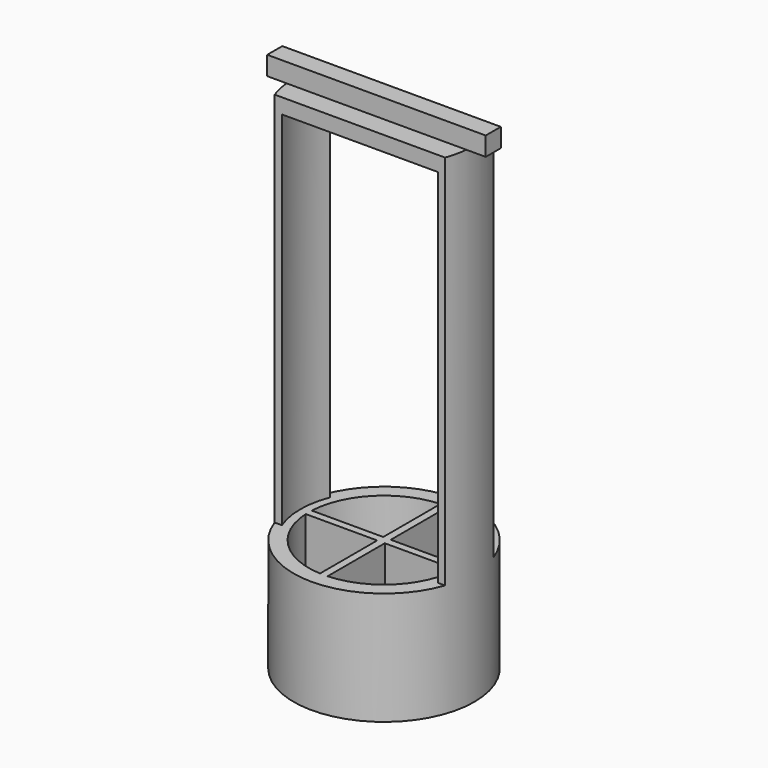
from build123d import *

# Parameters (mm, degrees)
F0_R      = 12
F1_DEPTH  = 15
F3_DEPTH  = 13
F4_R      = 12
F4_R_2    = 11.1
F5_DEPTH  = 50
F7_DEPTH  = 50
F8_W      = 22.627416998
F8_H      = 8
F9_DEPTH  = 2
F10_W     = 29
F10_H     = 2.5
F11_DEPTH = 2.5


with BuildPart() as f1:
    # F0 (on Top) → F1 (new body)
    with BuildSketch(Plane.XY):
        Circle(F0_R)
    extrude(amount=F1_DEPTH)

    # F2 (on face) → F3 (cut)
    with BuildSketch(Plane.XY.offset(15)):
        with BuildLine():
            Line((-0.5, 0.5), (-0.5, 9.9874921777))
            ThreePointArc((-0.5, 9.9874921777), (-7.0710678119, 7.0710678119), (-9.9874921777, 0.5))
            Line((-9.9874921777, 0.5), (-0.5, 0.5))
        make_face()
        with BuildLine():
            Line((0.5, 0.5), (9.9874921777, 0.5))
            ThreePointArc((9.9874921777, 0.5), (7.0710678119, 7.0710678119), (0.5, 9.9874921777))
            Line((0.5, 9.9874921777), (0.5, 0.5))
        make_face()
        with BuildLine():
            ThreePointArc((0.5, -9.9874921777), (7.0710678119, -7.0710678119), (9.9874921777, -0.5))
            Line((9.9874921777, -0.5), (0.5, -0.5))
            Line((0.5, -0.5), (0.5, -9.9874921777))
        make_face()
        with BuildLine():
            ThreePointArc((-9.9874921777, -0.5), (-7.0710678119, -7.0710678119), (-0.5, -9.9874921777))
            Line((-0.5, -9.9874921777), (-0.5, -0.5))
            Line((-0.5, -0.5), (-9.9874921777, -0.5))
        make_face()
    extrude(amount=-F3_DEPTH, mode=Mode.SUBTRACT)

    # F4 (on face) → F5 (join)
    with BuildSketch(Plane.XY.offset(15)):
        Circle(F4_R)
        Circle(F4_R_2, mode=Mode.SUBTRACT)
    extrude(amount=F5_DEPTH)

    # F6 (on face) → F7 (cut)
    with BuildSketch(Plane.XY.offset(65)):
        with BuildLine():
            Line((14.9746745975, -4), (14.8116537966, -4))
            Line((14.8116537966, -4), (11.313708499, -4))
            ThreePointArc((11.313708499, -4), (0, -12), (-11.313708499, -4))
            Line((-11.313708499, -4), (-14.8116537966, -4))
            Line((-14.8116537966, -4), (-14.8116537966, -14.8480758196))
            Line((-14.8116537966, -14.8480758196), (14.9746745975, -14.8480758196))
            Line((14.9746745975, -14.8480758196), (14.9746745975, -4))
        make_face()
        with BuildLine():
            Line((11.313708499, -4), (14.8116537966, -4))
            Line((14.8116537966, -4), (14.8116537966, 4))
            Line((14.8116537966, 4), (11.313708499, 4))
            ThreePointArc((11.313708499, 4), (11.8271827158, 2.0292237447), (12, 0))
            ThreePointArc((12, 0), (11.8271827158, -2.0292237447), (11.313708499, -4))
        make_face()
        with BuildLine():
            ThreePointArc((-11.313708499, -4), (0, -12), (11.313708499, -4))
            Line((11.313708499, -4), (10.3542261903, -4))
            ThreePointArc((10.3542261903, -4), (0, -11.1), (-10.3542261903, -4))
            Line((-10.3542261903, -4), (-11.313708499, -4))
        make_face()
        with BuildLine():
            Line((11.313708499, 4), (14.8116537966, 4))
            Line((14.8116537966, 4), (15.4569065875, 4))
            Line((15.4569065875, 4), (15.4569065875, 13.0318450025))
            Line((15.4569065875, 13.0318450025), (-14.8116537966, 13.0318450025))
            Line((-14.8116537966, 13.0318450025), (-14.8116537966, 4))
            Line((-14.8116537966, 4), (-11.313708499, 4))
            ThreePointArc((-11.313708499, 4), (0, 12), (11.313708499, 4))
        make_face()
        with BuildLine():
            Line((-10.3542261903, -4), (10.3542261903, -4))
            ThreePointArc((10.3542261903, -4), (10.9119638634, -2.0344642154), (11.1, 0))
            ThreePointArc((11.1, 0), (10.9119638634, 2.0344642154), (10.3542261903, 4))
            Line((10.3542261903, 4), (-10.3542261903, 4))
            ThreePointArc((-10.3542261903, 4), (-11.1, 0), (-10.3542261903, -4))
        make_face()
        with BuildLine():
            Line((10.3542261903, 4), (11.313708499, 4))
            ThreePointArc((11.313708499, 4), (0, 12), (-11.313708499, 4))
            Line((-11.313708499, 4), (-10.3542261903, 4))
            ThreePointArc((-10.3542261903, 4), (0, 11.1), (10.3542261903, 4))
        make_face()
    extrude(amount=-F7_DEPTH, mode=Mode.SUBTRACT)

    # F8 (on face) → F9 (join)
    with BuildSketch(Plane.XY.offset(65)):
        Rectangle(F8_W, F8_H)
    extrude(amount=-F9_DEPTH)

    # F10 (on face) → F11 (join)
    with BuildSketch(Plane.XY.offset(65)):
        Rectangle(F10_W, F10_H)
    extrude(amount=F11_DEPTH)


solid = f1.part
